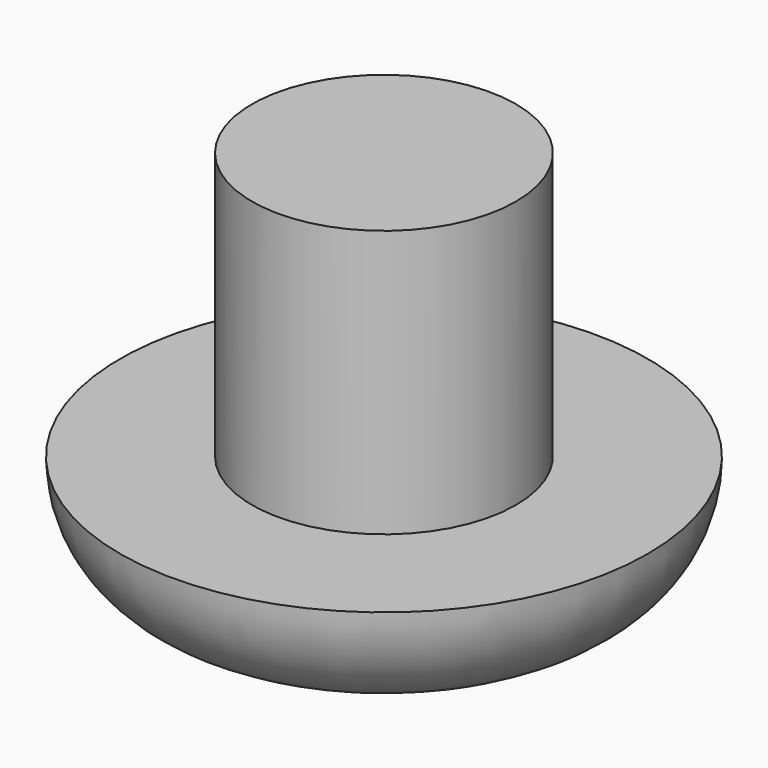
from build123d import *

# Parameters (mm, degrees)
F0_R     = 11.43
F1_DEPTH = 5.08
F2_R     = 5.07999
F3_R     = 5.715
F4_DEPTH = 11.5697


# Not quite as in the source:
# - a fillet or chamfer is up to 0.001 mm smaller than in the source, because OpenCascade refuses the exact size


with BuildPart() as f1:
    # F0 (on Top) → F1 (new body)
    with BuildSketch(Plane.XY):
        Circle(F0_R)
    extrude(amount=F1_DEPTH)

    # F2 (radius 5.08 in the source; OpenCascade refuses exactly that, so slightly less here)
    f2_edges = [f1.edges().sort_by_distance(p)[0] for p in [
        (-11.43, 0, 0),
    ]]
    fillet(f2_edges, radius=F2_R)

    # F3 (on face) → F4 (join)
    with BuildSketch(Plane.XY.offset(5.08)):
        Circle(F3_R)
    extrude(amount=F4_DEPTH)


solid = f1.part
